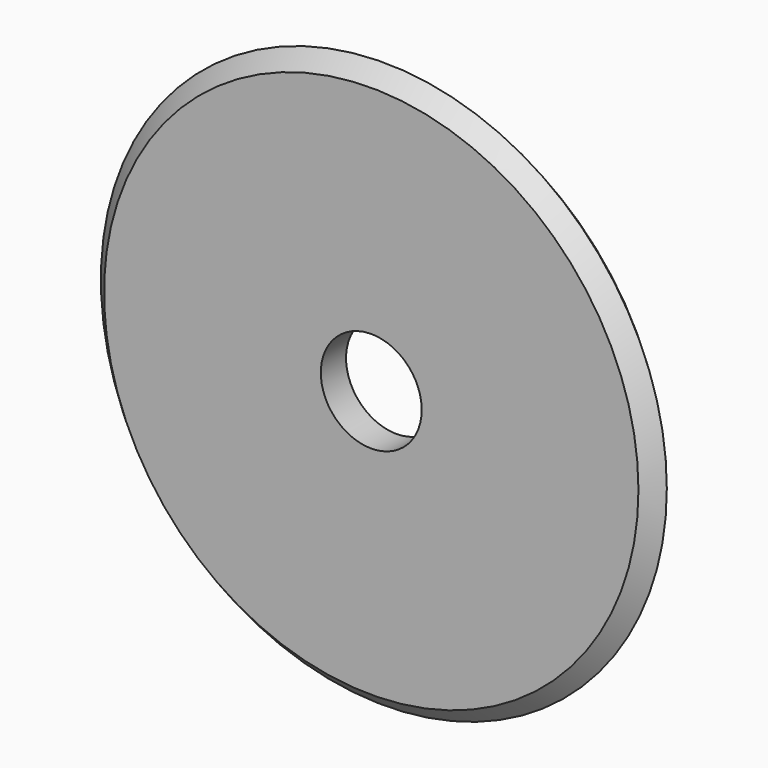
from build123d import *

# Parameters (mm, degrees)
F0_R     = 57.0036586855
F0_R_2   = 10.16
F1_DEPTH = 3.175
F2_SIZE  = 3.175
F3_SIZE  = 3.17499


# Not quite as in the source:
# - a fillet or chamfer is up to 0.001 mm smaller than in the source, because OpenCascade refuses the exact size


with BuildPart() as f1:
    # F0 (on Front) → F1 (new body, symmetric)
    with BuildSketch(Plane.XZ):
        Circle(F0_R)
        Circle(F0_R_2, mode=Mode.SUBTRACT)
    extrude(amount=F1_DEPTH, both=True)

    # F2
    f2_edges = [f1.edges().sort_by_distance(p)[0] for p in [
        (-57.003659, 3.175, 0),
    ]]
    chamfer(f2_edges, length=F2_SIZE)

    # F3 (size 3.175 in the source; OpenCascade refuses exactly that, so slightly less here)
    f3_edges = [f1.edges().sort_by_distance(p)[0] for p in [
        (-57.003659, -3.175, 0),
    ]]
    chamfer(f3_edges, length=F3_SIZE)


solid = f1.part
